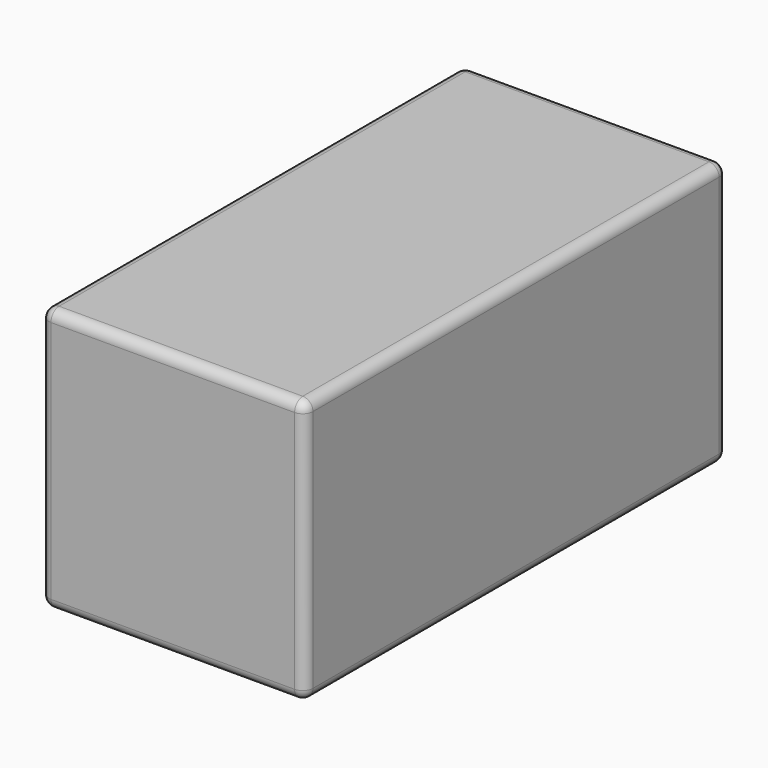
from build123d import *

# Parameters (mm, degrees)
F0_W         = 88.9
F0_H         = 88.9
F0_W_2       = 57.15
F0_H_2       = 57.15
F1_DEPTH     = 177.8
F2_DEPTH     = 15.875
F3_R         = 3.429
F4_T1_DEPTH  = 57.15
F4_T3_DEPTH  = 57.15
F4_T9_DEPTH  = 97.975467434
F4_T13_DEPTH = 97.975467434
F4_T20_DEPTH = 97.975467434
F4_T24_DEPTH = 97.975467434
F4_T31_DEPTH = 97.975467434
F4_T35_DEPTH = 97.975467434
F4_T42_DEPTH = 97.975467434
F4_T46_DEPTH = 97.975467434


# Not quite as in the source:
# - a fillet or chamfer that OpenCascade refuses, or shapes differently, is made with other operations: its cross-section is extruded or revolved along the edge and cut away or added


with BuildPart() as f1:
    # F0 (on Front) → F1 (new body)
    with BuildSketch(Plane.XZ):
        Rectangle(F0_W, F0_H)
        Rectangle(F0_W_2, F0_H_2, mode=Mode.SUBTRACT)
    extrude(amount=-F1_DEPTH)

    # F0 (on Front) → F2 (join)
    with BuildSketch(Plane.XZ):
        Rectangle(F0_W, F0_H)
        Rectangle(F0_W_2, F0_H_2, mode=Mode.SUBTRACT)
        Rectangle(F0_W_2, F0_H_2)
    extrude(amount=-F2_DEPTH)

    # F3
    f3_edges = [f1.edges().sort_by_distance(p)[0] for p in [
        (44.45, 88.9, 44.45),
        (0, 0, 44.45),
        (44.45, 0, 0),
        (0, 0, -44.45),
        (44.45, 88.9, -44.45),
        (-44.45, 0, 0),
        (-44.45, 88.9, -44.45),
        (0, 177.8, 44.45),
        (-44.45, 88.9, 44.45),
        (-44.45, 177.8, 0),
        (0, 177.8, -44.45),
        (44.45, 177.8, 0),
    ]]
    fillet(f3_edges, radius=F3_R)

    # F4: chamfer of 15.875 on 4 edges, made by hand

    # F4_s2 → F4_t1 (cut)
    with BuildSketch(Plane.XY.offset(-28.575)):
        with BuildLine():
            Line((-44.8990128061, 178.2490128061), (-28.1259871939, 161.4759871939))
            Line((-28.1259871939, 161.4759871939), (-27.8084871939, 161.4759871939))
            ThreePointArc((-27.8084871939, 161.4759871939), (-28.2575, 169.637993597), (-28.2575, 177.8))
            Line((-28.2575, 177.8), (-28.575, 178.1175))
            ThreePointArc((-28.575, 178.1175), (-36.737006403, 178.1175), (-44.8990128061, 178.5665128061))
            Line((-44.8990128061, 178.5665128061), (-44.8990128061, 178.2490128061))
        make_face()
        with BuildLine():
            Line((44.8990128061, 178.2490128061), (28.1259871939, 161.4759871939))
            Line((28.1259871939, 161.4759871939), (27.8084871939, 161.4759871939))
            ThreePointArc((27.8084871939, 161.4759871939), (28.2575, 169.637993597), (28.2575, 177.8))
            Line((28.2575, 177.8), (28.575, 178.1175))
            ThreePointArc((28.575, 178.1175), (36.737006403, 178.1175), (44.8990128061, 178.5665128061))
            Line((44.8990128061, 178.5665128061), (44.8990128061, 178.2490128061))
        make_face()
    extrude(amount=F4_T1_DEPTH, mode=Mode.SUBTRACT)

    # F4_s4 → F4_t3 (cut)
    with BuildSketch(Plane.YZ.offset(-28.575)):
        with BuildLine():
            Line((178.2490128061, -44.8990128061), (161.4759871939, -28.1259871939))
            Line((161.4759871939, -28.1259871939), (161.4759871939, -27.8084871939))
            ThreePointArc((161.4759871939, -27.8084871939), (169.637993597, -28.2575), (177.8, -28.2575))
            Line((177.8, -28.2575), (178.1175, -28.575))
            ThreePointArc((178.1175, -28.575), (178.1175, -36.737006403), (178.5665128061, -44.8990128061))
            Line((178.5665128061, -44.8990128061), (178.2490128061, -44.8990128061))
        make_face()
        with BuildLine():
            Line((178.2490128061, 44.8990128061), (161.4759871939, 28.1259871939))
            Line((161.4759871939, 28.1259871939), (161.4759871939, 27.8084871939))
            ThreePointArc((161.4759871939, 27.8084871939), (169.637993597, 28.2575), (177.8, 28.2575))
            Line((177.8, 28.2575), (178.1175, 28.575))
            ThreePointArc((178.1175, 28.575), (178.1175, 36.737006403), (178.5665128061, 44.8990128061))
            Line((178.5665128061, 44.8990128061), (178.2490128061, 44.8990128061))
        make_face()
    extrude(amount=F4_T3_DEPTH, mode=Mode.SUBTRACT)


with BuildPart() as f4_tool7:
    # F4_s8 → F4_t9 (new body)
    with BuildSketch(Plane.XY.offset(-69.400467434)):
        with BuildLine():
            Line((-44.8990128061, 178.2490128061), (-28.1259871939, 161.4759871939))
            Line((-28.1259871939, 161.4759871939), (-27.8084871939, 161.4759871939))
            ThreePointArc((-27.8084871939, 161.4759871939), (-28.2575, 169.637993597), (-28.2575, 177.8))
            Line((-28.2575, 177.8), (-28.575, 178.1175))
            ThreePointArc((-28.575, 178.1175), (-36.737006403, 178.1175), (-44.8990128061, 178.5665128061))
            Line((-44.8990128061, 178.5665128061), (-44.8990128061, 178.2490128061))
        make_face()
    extrude(amount=F4_T9_DEPTH)

    split(bisect_by=Plane.XY.offset(-28.575), keep=Keep.BOTTOM)


with BuildPart() as f4_tool11:
    # F4_s12 → F4_t13 (new body)
    with BuildSketch(Plane.YZ.offset(28.575)):
        with BuildLine():
            Line((178.2490128061, -44.8990128061), (161.4759871939, -28.1259871939))
            Line((161.4759871939, -28.1259871939), (161.4759871939, -27.8084871939))
            ThreePointArc((161.4759871939, -27.8084871939), (169.637993597, -28.2575), (177.8, -28.2575))
            Line((177.8, -28.2575), (178.1175, -28.575))
            ThreePointArc((178.1175, -28.575), (178.1175, -36.737006403), (178.5665128061, -44.8990128061))
            Line((178.5665128061, -44.8990128061), (178.2490128061, -44.8990128061))
        make_face()
    extrude(amount=-F4_T13_DEPTH)

    split(bisect_by=Plane.YZ.offset(-28.575), keep=Keep.BOTTOM)


with BuildPart() as f4_tool7_1:
    add(f4_tool7.part)

    # F4_t15: intersect F4_tool11
    add(f4_tool11.part, mode=Mode.INTERSECT)


with BuildPart() as f1_1:
    add(f1.part)

    # F4_t5: cut F4_tool7
    add(f4_tool7_1.part, mode=Mode.SUBTRACT)


with BuildPart() as f4_tool18:
    # F4_s19 → F4_t20 (new body)
    with BuildSketch(Plane.XY.offset(-28.575)):
        with BuildLine():
            Line((-44.8990128061, 178.2490128061), (-28.1259871939, 161.4759871939))
            Line((-28.1259871939, 161.4759871939), (-27.8084871939, 161.4759871939))
            ThreePointArc((-27.8084871939, 161.4759871939), (-28.2575, 169.637993597), (-28.2575, 177.8))
            Line((-28.2575, 177.8), (-28.575, 178.1175))
            ThreePointArc((-28.575, 178.1175), (-36.737006403, 178.1175), (-44.8990128061, 178.5665128061))
            Line((-44.8990128061, 178.5665128061), (-44.8990128061, 178.2490128061))
        make_face()
    extrude(amount=F4_T20_DEPTH)

    split(bisect_by=Plane.XY.offset(28.575), keep=Keep.TOP)


with BuildPart() as f4_tool22:
    # F4_s23 → F4_t24 (new body)
    with BuildSketch(Plane.YZ.offset(-69.400467434)):
        with BuildLine():
            Line((178.2490128061, 44.8990128061), (161.4759871939, 28.1259871939))
            Line((161.4759871939, 28.1259871939), (161.4759871939, 27.8084871939))
            ThreePointArc((161.4759871939, 27.8084871939), (169.637993597, 28.2575), (177.8, 28.2575))
            Line((177.8, 28.2575), (178.1175, 28.575))
            ThreePointArc((178.1175, 28.575), (178.1175, 36.737006403), (178.5665128061, 44.8990128061))
            Line((178.5665128061, 44.8990128061), (178.2490128061, 44.8990128061))
        make_face()
    extrude(amount=F4_T24_DEPTH)

    split(bisect_by=Plane.YZ.offset(-28.575), keep=Keep.BOTTOM)


with BuildPart() as f4_tool18_1:
    add(f4_tool18.part)

    # F4_t26: intersect F4_tool22
    add(f4_tool22.part, mode=Mode.INTERSECT)


with BuildPart() as f1_2:
    add(f1_1.part)

    # F4_t16: cut F4_tool18
    add(f4_tool18_1.part, mode=Mode.SUBTRACT)


with BuildPart() as f4_tool29:
    # F4_s30 → F4_t31 (new body)
    with BuildSketch(Plane.XY.offset(28.575)):
        with BuildLine():
            Line((44.8990128061, 178.2490128061), (28.1259871939, 161.4759871939))
            Line((28.1259871939, 161.4759871939), (27.8084871939, 161.4759871939))
            ThreePointArc((27.8084871939, 161.4759871939), (28.2575, 169.637993597), (28.2575, 177.8))
            Line((28.2575, 177.8), (28.575, 178.1175))
            ThreePointArc((28.575, 178.1175), (36.737006403, 178.1175), (44.8990128061, 178.5665128061))
            Line((44.8990128061, 178.5665128061), (44.8990128061, 178.2490128061))
        make_face()
    extrude(amount=-F4_T31_DEPTH)

    split(bisect_by=Plane.XY.offset(-28.575), keep=Keep.BOTTOM)


with BuildPart() as f4_tool33:
    # F4_s34 → F4_t35 (new body)
    with BuildSketch(Plane.YZ.offset(69.400467434)):
        with BuildLine():
            Line((178.2490128061, -44.8990128061), (161.4759871939, -28.1259871939))
            Line((161.4759871939, -28.1259871939), (161.4759871939, -27.8084871939))
            ThreePointArc((161.4759871939, -27.8084871939), (169.637993597, -28.2575), (177.8, -28.2575))
            Line((177.8, -28.2575), (178.1175, -28.575))
            ThreePointArc((178.1175, -28.575), (178.1175, -36.737006403), (178.5665128061, -44.8990128061))
            Line((178.5665128061, -44.8990128061), (178.2490128061, -44.8990128061))
        make_face()
    extrude(amount=-F4_T35_DEPTH)

    split(bisect_by=Plane.YZ.offset(28.575), keep=Keep.TOP)


with BuildPart() as f4_tool29_1:
    add(f4_tool29.part)

    # F4_t37: intersect F4_tool33
    add(f4_tool33.part, mode=Mode.INTERSECT)


with BuildPart() as f1_3:
    add(f1_2.part)

    # F4_t27: cut F4_tool29
    add(f4_tool29_1.part, mode=Mode.SUBTRACT)


with BuildPart() as f4_tool40:
    # F4_s41 → F4_t42 (new body)
    with BuildSketch(Plane.YZ.offset(-28.575)):
        with BuildLine():
            Line((178.2490128061, 44.8990128061), (161.4759871939, 28.1259871939))
            Line((161.4759871939, 28.1259871939), (161.4759871939, 27.8084871939))
            ThreePointArc((161.4759871939, 27.8084871939), (169.637993597, 28.2575), (177.8, 28.2575))
            Line((177.8, 28.2575), (178.1175, 28.575))
            ThreePointArc((178.1175, 28.575), (178.1175, 36.737006403), (178.5665128061, 44.8990128061))
            Line((178.5665128061, 44.8990128061), (178.2490128061, 44.8990128061))
        make_face()
    extrude(amount=F4_T42_DEPTH)

    split(bisect_by=Plane.YZ.offset(28.575), keep=Keep.TOP)


with BuildPart() as f4_tool44:
    # F4_s45 → F4_t46 (new body)
    with BuildSketch(Plane.XY.offset(69.400467434)):
        with BuildLine():
            Line((44.8990128061, 178.2490128061), (28.1259871939, 161.4759871939))
            Line((28.1259871939, 161.4759871939), (27.8084871939, 161.4759871939))
            ThreePointArc((27.8084871939, 161.4759871939), (28.2575, 169.637993597), (28.2575, 177.8))
            Line((28.2575, 177.8), (28.575, 178.1175))
            ThreePointArc((28.575, 178.1175), (36.737006403, 178.1175), (44.8990128061, 178.5665128061))
            Line((44.8990128061, 178.5665128061), (44.8990128061, 178.2490128061))
        make_face()
    extrude(amount=-F4_T46_DEPTH)

    split(bisect_by=Plane.XY.offset(28.575), keep=Keep.TOP)


with BuildPart() as f4_tool40_1:
    add(f4_tool40.part)

    # F4_t48: intersect F4_tool44
    add(f4_tool44.part, mode=Mode.INTERSECT)


with BuildPart() as f1_4:
    add(f1_3.part)

    # F4_t38: cut F4_tool40
    add(f4_tool40_1.part, mode=Mode.SUBTRACT)


solid = f1_4.part
